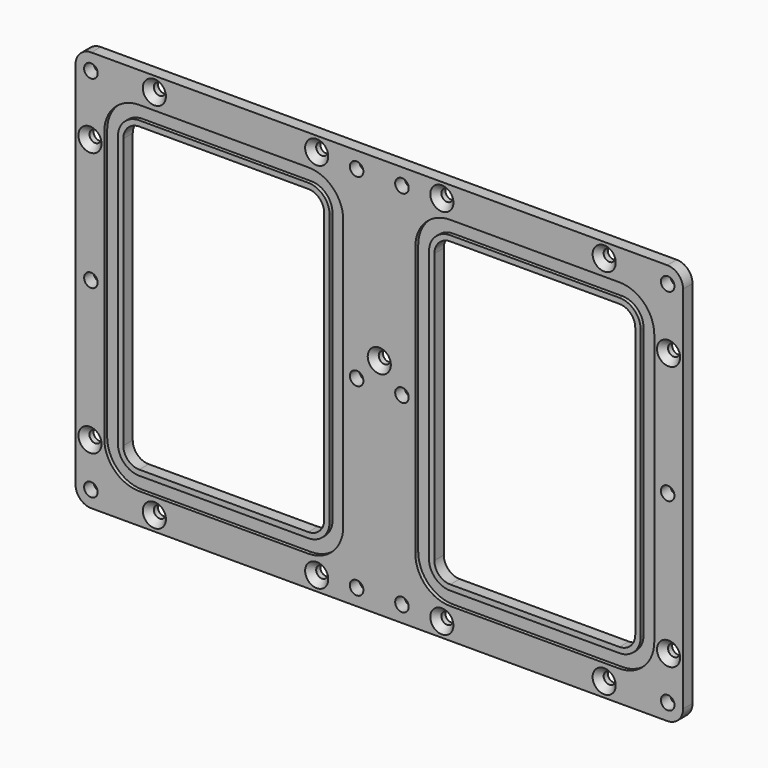
from build123d import *

# Parameters (mm, degrees)
F1_DEPTH       = 3.302
F3_DEPTH       = 1.016
F6_D           = 3.2639
F6_CSINK_D     = 6.477
F6_CSINK_ANGLE = 82
F8_D           = 3.7973


# Not quite as in the source:
# - a pattern or mirror of a feature is missing from the dataset's text; its kind, count and spacing are read off the source's solid


with BuildPart() as f1:
    # F0 (on Front) → F1 (new body)
    with BuildSketch(Plane.XZ):
        with BuildLine():
            ThreePointArc((-85.09, -51.7525), (-83.7880896424, -54.8955896424), (-80.645, -56.1975))
            Line((-80.645, -56.1975), (80.645, -56.1975))
            ThreePointArc((80.645, -56.1975), (83.7880896424, -54.8955896424), (85.09, -51.7525))
            Line((85.09, -51.7525), (85.09, 51.7525))
            ThreePointArc((85.09, 51.7525), (83.7880896424, 54.8955896424), (80.645, 56.1975))
            Line((80.645, 56.1975), (-80.645, 56.1975))
            ThreePointArc((-80.645, 56.1975), (-83.7880896424, 54.8955896424), (-85.09, 51.7525))
            Line((-85.09, 51.7525), (-85.09, -51.7525))
        make_face()
        with BuildLine():
            ThreePointArc((-15.4305, -37.846), (-16.7324103576, -40.9890896424), (-19.8755, -42.291))
            Line((-19.8755, -42.291), (-67.2465, -42.291))
            ThreePointArc((-67.2465, -42.291), (-70.3895896424, -40.9890896424), (-71.6915, -37.846))
            Line((-71.6915, -37.846), (-71.6915, 37.846))
            ThreePointArc((-71.6915, 37.846), (-70.3895896424, 40.9890896424), (-67.2465, 42.291))
            Line((-67.2465, 42.291), (-19.8755, 42.291))
            ThreePointArc((-19.8755, 42.291), (-16.7324103576, 40.9890896424), (-15.4305, 37.846))
            Line((-15.4305, 37.846), (-15.4305, -37.846))
        make_face(mode=Mode.SUBTRACT)
        with BuildLine():
            Line((19.8755, 42.291), (67.2465, 42.291))
            ThreePointArc((67.2465, 42.291), (70.3895896424, 40.9890896424), (71.6915, 37.846))
            Line((71.6915, 37.846), (71.6915, -37.846))
            ThreePointArc((71.6915, -37.846), (70.3895896424, -40.9890896424), (67.2465, -42.291))
            Line((67.2465, -42.291), (19.8755, -42.291))
            ThreePointArc((19.8755, -42.291), (16.7324103576, -40.9890896424), (15.4305, -37.846))
            Line((15.4305, -37.846), (15.4305, 37.846))
            ThreePointArc((15.4305, 37.846), (16.7324103576, 40.9890896424), (19.8755, 42.291))
        make_face(mode=Mode.SUBTRACT)
    extrude(amount=F1_DEPTH)

    # F2 (on face) → F3 (cut)
    with BuildSketch(Plane.XZ.offset(3.302)):
        with BuildLine():
            ThreePointArc((-10.0965, 37.846), (-12.9607027868, 44.7607972132), (-19.8755, 47.625))
            Line((-19.8755, 47.625), (-67.2465, 47.625))
            ThreePointArc((-67.2465, 47.625), (-74.1612972132, 44.7607972132), (-77.0255, 37.846))
            Line((-77.0255, 37.846), (-77.0255, -37.846))
            ThreePointArc((-77.0255, -37.846), (-74.1612972132, -44.7607972132), (-67.2465, -47.625))
            Line((-67.2465, -47.625), (-19.8755, -47.625))
            ThreePointArc((-19.8755, -47.625), (-12.9607027868, -44.7607972132), (-10.0965, -37.846))
            Line((-10.0965, -37.846), (-10.0965, 37.846))
        make_face()
        with BuildLine():
            ThreePointArc((-19.8755, 43.815), (-15.6547796231, 42.0667203769), (-13.9065, 37.846))
            Line((-13.9065, 37.846), (-13.9065, -37.846))
            ThreePointArc((-13.9065, -37.846), (-15.6547796231, -42.0667203769), (-19.8755, -43.815))
            Line((-19.8755, -43.815), (-67.2465, -43.815))
            ThreePointArc((-67.2465, -43.815), (-71.4672203769, -42.0667203769), (-73.2155, -37.846))
            Line((-73.2155, -37.846), (-73.2155, 37.846))
            ThreePointArc((-73.2155, 37.846), (-71.4672203769, 42.0667203769), (-67.2465, 43.815))
            Line((-67.2465, 43.815), (-19.8755, 43.815))
        make_face(mode=Mode.SUBTRACT)
        with BuildLine():
            ThreePointArc((10.0965, -37.846), (12.9607027868, -44.7607972132), (19.8755, -47.625))
            Line((19.8755, -47.625), (67.2465, -47.625))
            ThreePointArc((67.2465, -47.625), (74.1612972132, -44.7607972132), (77.0255, -37.846))
            Line((77.0255, -37.846), (77.0255, 37.846))
            ThreePointArc((77.0255, 37.846), (74.1612972132, 44.7607972132), (67.2465, 47.625))
            Line((67.2465, 47.625), (19.8755, 47.625))
            ThreePointArc((19.8755, 47.625), (12.9607027868, 44.7607972132), (10.0965, 37.846))
            Line((10.0965, 37.846), (10.0965, -37.846))
        make_face()
        with BuildLine():
            Line((73.2155, 37.846), (73.2155, -37.846))
            ThreePointArc((73.2155, -37.846), (71.4672203769, -42.0667203769), (67.2465, -43.815))
            Line((67.2465, -43.815), (19.8755, -43.815))
            ThreePointArc((19.8755, -43.815), (15.6547796231, -42.0667203769), (13.9065, -37.846))
            Line((13.9065, -37.846), (13.9065, 37.846))
            ThreePointArc((13.9065, 37.846), (15.6547796231, 42.0667203769), (19.8755, 43.815))
            Line((19.8755, 43.815), (67.2465, 43.815))
            ThreePointArc((67.2465, 43.815), (71.4672203769, 42.0667203769), (73.2155, 37.846))
        make_face(mode=Mode.SUBTRACT)
    f3 = extrude(amount=-F3_DEPTH, mode=Mode.SUBTRACT)

    # F3_copies: F3 across plane
    add(f3.mirror(Plane.ZX.offset(-1.651)), mode=Mode.SUBTRACT)

    # F6 (through all)
    with Locations(Plane.XZ.offset(3.302)):
        with Locations((-81.026, 34.6075), (-81.026, -39.4335), (-62.992, 52.1335), (-17.526, 52.1335), (0, 6.4135), (-62.992, -52.1335), (-17.526, -52.1335), (17.526, -52.1335), (62.992, -52.1335), (81.026, -39.4335), (81.026, 34.6075), (62.992, 52.1335), (17.526, 52.1335)):
            CounterSinkHole(F6_D / 2, F6_CSINK_D / 2, counter_sink_angle=F6_CSINK_ANGLE)

    # F8 (through all)
    with Locations(Plane.XZ.offset(3.302)):
        with Locations((-80.772, 51.6255), (-80.772, 0), (-80.772, -51.6255), (-6.35, -51.6255), (-6.35, 0), (6.35, 0), (-6.35, 51.6255), (6.35, 51.6255), (6.35, -51.6255), (80.772, -51.6255), (80.772, 51.6255), (80.772, 0)):
            Hole(F8_D / 2)


solid = f1.part
